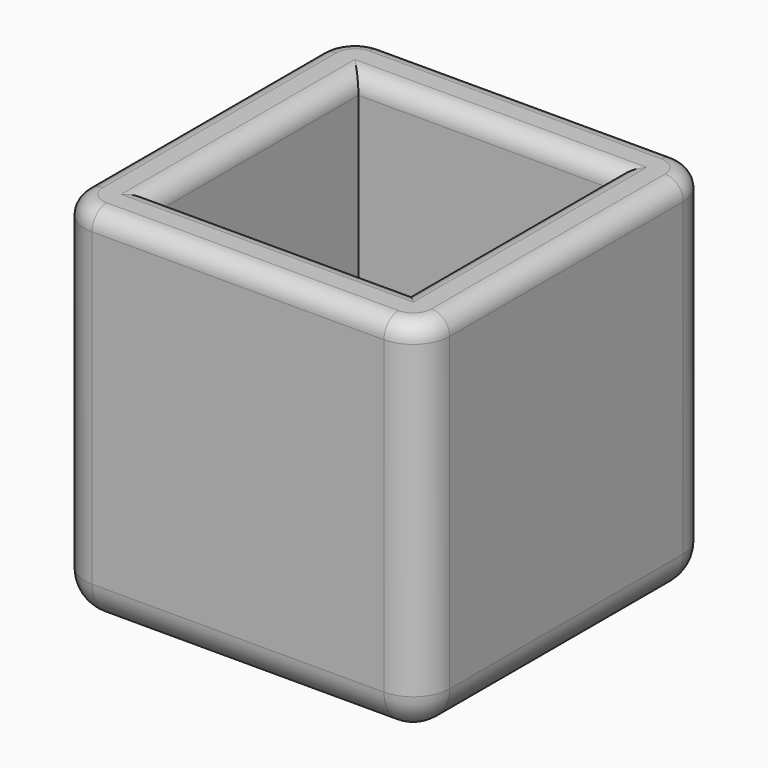
from build123d import *

# Parameters (mm, degrees)
F1_DEPTH = 20
F2_R     = 2
F3_T     = -3
F4_R     = 1
F5_R     = 2


with BuildPart() as f1:
    # F0 (on Top) → F1 (new body)
    with BuildSketch(Plane.XY):
        with BuildLine():
            Line((8, 10), (-8, 10))
            ThreePointArc((-8, 10), (-9.4142135624, 9.4142135624), (-10, 8))
            Line((-10, 8), (-10, -8))
            ThreePointArc((-10, -8), (-9.4142135624, -9.4142135624), (-8, -10))
            Line((-8, -10), (8, -10))
            ThreePointArc((8, -10), (9.4142135624, -9.4142135624), (10, -8))
            Line((10, -8), (10, 8))
            ThreePointArc((10, 8), (9.4142135624, 9.4142135624), (8, 10))
        make_face()
    extrude(amount=F1_DEPTH)

    # F2
    f2_edges = [f1.edges().sort_by_distance(p)[0] for p in [
        (0, -10, 0),
    ]]
    fillet(f2_edges, radius=F2_R)

    # F3
    f3_openings = [f1.faces().sort_by_distance(p)[0] for p in [
        (0, 0, 20),
    ]]
    offset(amount=F3_T, openings=f3_openings)

    # F4
    f4_edges = [f1.edges().sort_by_distance(p)[0] for p in [
        (-10, 0, 20),
        (7, 0, 20),
        (0, 7, 20),
        (-7, 0, 20),
        (0, -7, 20),
        (0, 10, 20),
        (9.414214, 9.414214, 20),
        (-9.414214, 9.414214, 20),
        (10, 0, 20),
        (-9.414214, -9.414214, 20),
        (0, -10, 20),
        (9.414214, -9.414214, 20),
    ]]
    fillet(f4_edges, radius=F4_R)

    # F5
    f5_edges = [f1.edges().sort_by_distance(p)[0] for p in [
        (7, 0, 3),
        (0, -7, 3),
        (0, 7, 3),
        (-7, 0, 3),
    ]]
    fillet(f5_edges, radius=F5_R)


solid = f1.part
